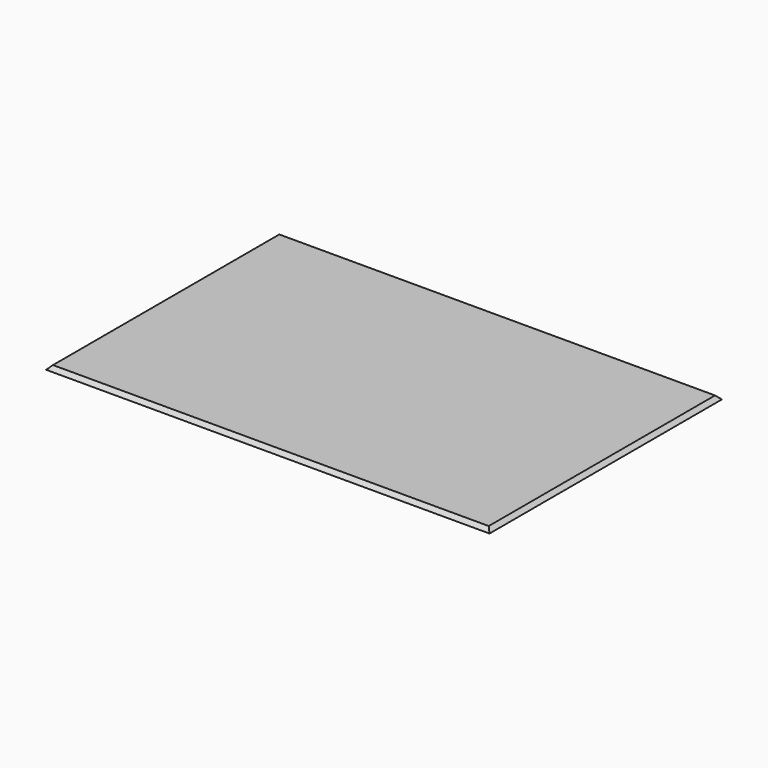
from build123d import *

# Parameters (mm, degrees)
F0_W     = 580
F0_H     = 380
F1_DEPTH = 5
F2_SIZE  = 4.99999


# Not quite as in the source:
# - a fillet or chamfer is up to 0.001 mm smaller than in the source, because OpenCascade refuses the exact size


with BuildPart() as f1:
    # F0 (on Top) → F1 (new body)
    with BuildSketch(Plane.XY):
        Rectangle(F0_W, F0_H)
    extrude(amount=F1_DEPTH)

    # F2 (size 5 in the source; OpenCascade refuses exactly that, so slightly less here)
    f2_edges = [f1.edges().sort_by_distance(p)[0] for p in [
        (0, 190, 5),
        (-290, 0, 5),
        (0, -190, 5),
        (290, 0, 5),
    ]]
    chamfer(f2_edges, length=F2_SIZE)


solid = f1.part
